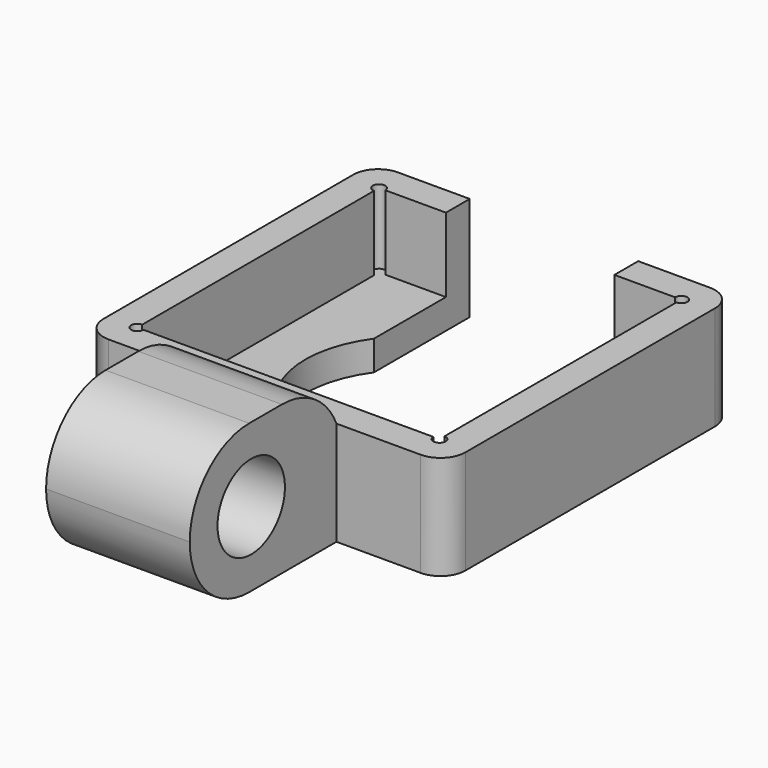
from build123d import *

# Parameters (mm, degrees)
F1_DEPTH    = 1.2
F2_DEPTH    = 4.2
F3_DEPTH    = 6
F6_T1_DEPTH = 20.8
F6_T3_DEPTH = 19.5477270849
F7_D        = 3.4
F7_DEPTH    = 7
F7_TIP      = 1.0214630523
F8_R        = 1


# Not quite as in the source:
# - a fillet or chamfer that OpenCascade refuses, or shapes differently, is made with other operations: its cross-section is extruded or revolved along the edge and cut away or added


with BuildPart() as f1:
    # F0 (on Top) → F1 (new body)
    with BuildSketch(Plane.XY):
        with BuildLine():
            Line((-3.4, 6.1), (-5.85, 6.1))
            ThreePointArc((-5.85, 6.1), (-6.2767766953, 6.2767766953), (-6.1, 5.85))
            Line((-6.1, 5.85), (-6.1, -5.85))
            ThreePointArc((-6.1, -5.85), (-6.2767766953, -6.2767766953), (-5.85, -6.1))
            Line((-5.85, -6.1), (5.85, -6.1))
            ThreePointArc((5.85, -6.1), (6.2767766953, -6.2767766953), (6.1, -5.85))
            Line((6.1, -5.85), (6.1, 5.85))
            ThreePointArc((6.1, 5.85), (6.2767766953, 6.2767766953), (5.85, 6.1))
            Line((5.85, 6.1), (3.4, 6.1))
            Line((3.4, 6.1), (3.4, 2.4657656012))
            ThreePointArc((3.4, 2.4657656012), (0, -4.2), (-3.4, 2.4657656012))
            Line((-3.4, 2.4657656012), (-3.4, 6.1))
        make_face()
    extrude(amount=F1_DEPTH)

    # F0 (on Top) → F2 (join)
    with BuildSketch(Plane.XY):
        with BuildLine():
            ThreePointArc((-6.1, 5.85), (-6.2767766953, 6.2767766953), (-5.85, 6.1))
            Line((-5.85, 6.1), (-3.4, 6.1))
            Line((-3.4, 6.1), (-3.4, 7.3))
            Line((-3.4, 7.3), (-7.3, 7.3))
            Line((-7.3, 7.3), (-7.3, -7.3))
            Line((-7.3, -7.3), (-2.9, -7.3))
            Line((-2.9, -7.3), (2.9, -7.3))
            Line((2.9, -7.3), (7.3, -7.3))
            Line((7.3, -7.3), (7.3, 7.3))
            Line((7.3, 7.3), (3.4, 7.3))
            Line((3.4, 7.3), (3.4, 6.1))
            Line((3.4, 6.1), (5.85, 6.1))
            ThreePointArc((5.85, 6.1), (6.2767766953, 6.2767766953), (6.1, 5.85))
            Line((6.1, 5.85), (6.1, -5.85))
            ThreePointArc((6.1, -5.85), (6.2767766953, -6.2767766953), (5.85, -6.1))
            Line((5.85, -6.1), (-5.85, -6.1))
            ThreePointArc((-5.85, -6.1), (-6.2767766953, -6.2767766953), (-6.1, -5.85))
            Line((-6.1, -5.85), (-6.1, 5.85))
        make_face()
    extrude(amount=F2_DEPTH)

    # F0 (on Top) → F3 (join)
    with BuildSketch(Plane.XY):
        Polygon((2.9, -7.3), (-2.9, -7.3), (-2.9, -14.7), (0, -14.7), (2.9, -14.7), align=None)
    extrude(amount=F3_DEPTH)

    # F6: fillet of radius 3 on 3 edges, made by hand

    # F6_s2 → F6_t1 (cut)
    with BuildSketch(Plane.YZ.offset(-10.4)):
        with BuildLine():
            ThreePointArc((-11.7, 0), (-13.8213203436, 0.8786796564), (-14.7, 3))
            Line((-14.7, 3), (-14.7, 0))
            Line((-14.7, 0), (-11.7, 0))
        make_face()
        with BuildLine():
            ThreePointArc((-11.7, 6), (-13.8213203436, 5.1213203436), (-14.7, 3))
            Line((-14.7, 3), (-14.7, 6))
            Line((-14.7, 6), (-11.7, 6))
        make_face()
    extrude(amount=F6_T1_DEPTH, mode=Mode.SUBTRACT)

    # F6_s4 → F6_t3 (cut)
    with BuildSketch(Plane.YZ.offset(-9.7738635424)):
        with BuildLine():
            ThreePointArc((-7.3, 4.2), (-8.4063777445, 5.5099800796), (-10.049545417, 6))
            Line((-10.049545417, 6), (-7.3, 6))
            Line((-7.3, 6), (-7.3, 4.2))
        make_face()
    extrude(amount=F6_T3_DEPTH, mode=Mode.SUBTRACT)

    # F7
    with Locations(Plane.YZ.offset(3)):
        with Locations((-11.6, 3)):
            Hole(F7_D / 2, depth=F7_DEPTH)
            with Locations((0, 0, -(F7_DEPTH + F7_TIP / 2))):  # 118° drill point
                Cone(0, F7_D / 2, F7_TIP, mode=Mode.SUBTRACT)

    # F8
    f8_edges = [f1.edges().sort_by_distance(p)[0] for p in [
        (-7.3, 7.3, 2.1),
        (-7.3, -7.3, 2.1),
        (7.3, 7.3, 2.1),
        (7.3, -7.3, 2.1),
    ]]
    fillet(f8_edges, radius=F8_R)


solid = f1.part
